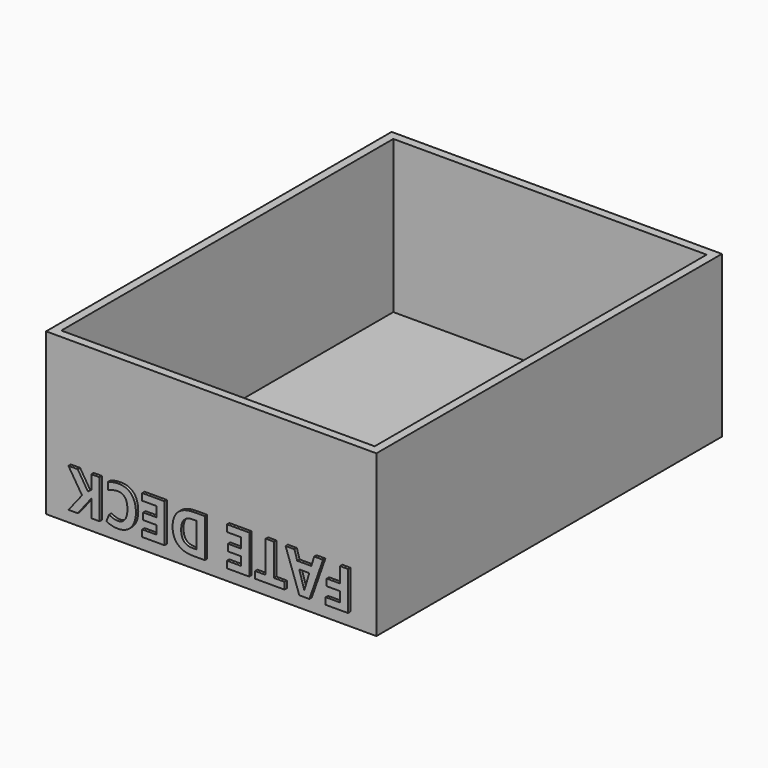
from build123d import *

# Parameters (mm, degrees)
F0_W         = 78
F0_H         = 102
F1_DEPTH     = 38
F2_W         = 74
F2_H         = 98
F3_DEPTH     = 36
F4_TEXT_SIZE = 12.8199840929
F5_DEPTH     = 0.7


# Not quite as in the source:
# - Text() gives the source's letters only with a copy of the font that has no kerning and outlines rounded to 1/6400 em; it was checked with that copy


with BuildPart() as f1:
    # F0 (on Top) → F1 (new body)
    with BuildSketch(Plane.XY):
        Rectangle(F0_W, F0_H)
    extrude(amount=F1_DEPTH)

    # F2 (on face) → F3 (cut)
    with BuildSketch(Plane.XY.offset(38)):
        Rectangle(F2_W, F2_H)
    extrude(amount=-F3_DEPTH, mode=Mode.SUBTRACT)

    # F4 (on face) → F5 (join)
    with BuildSketch(Plane.XZ.offset(51)):
        with Locations(Location((34, 12.2303885469), (0, 0, 180))):
            Text('FATE DECK', F4_TEXT_SIZE, font='Open Sans', font_style=FontStyle.BOLD, text_align=(TextAlign.LEFT, TextAlign.BOTTOM))
    extrude(amount=F5_DEPTH)


solid = f1.part
